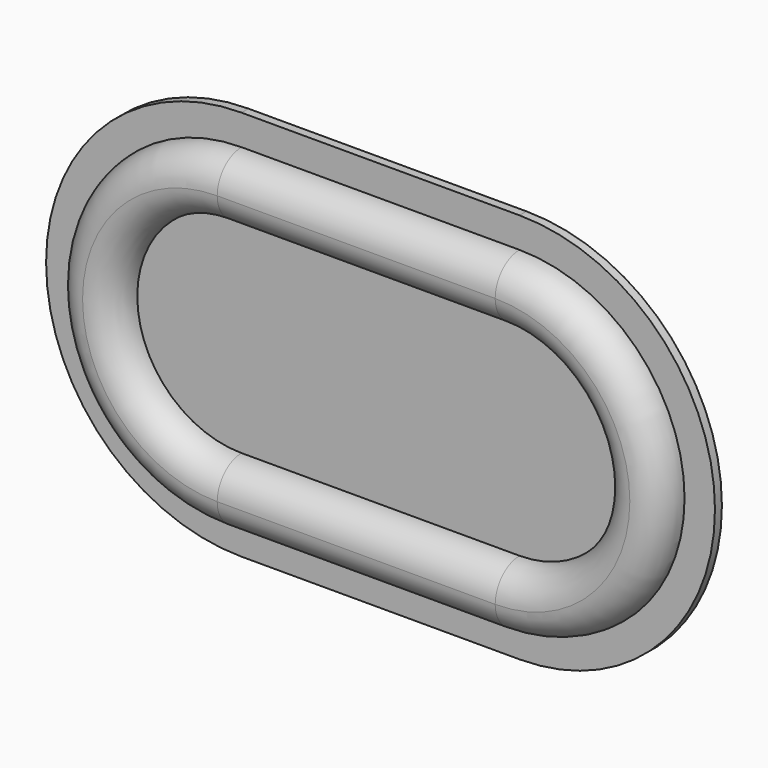
from build123d import *

# Parameters (mm, degrees)
F0_W     = 32
F0_H     = 45
F1_DEPTH = 1
F3_DEPTH = 3.5
F4_R     = 3.49999


# Not quite as in the source:
# - a fillet or chamfer is up to 0.001 mm smaller than in the source, because OpenCascade refuses the exact size


with BuildPart() as f1:
    # F0 (on Front) → F1 (new body)
    with BuildSketch(Plane.XZ):
        with BuildLine():
            Line((16, 22.5), (16, -22.5))
            ThreePointArc((16, -22.5), (38.5, 0), (16, 22.5))
        make_face()
        Rectangle(F0_W, F0_H)
        with BuildLine():
            ThreePointArc((-16, 22.5), (-38.5, 0), (-16, -22.5))
            Line((-16, -22.5), (-16, 22.5))
        make_face()
    extrude(amount=F1_DEPTH)

    # F2 (on face) → F3 (join)
    with BuildSketch(Plane.XZ.offset(1)):
        with BuildLine():
            ThreePointArc((16, -19), (35, 0), (16, 19))
            Line((16, 19), (-16, 19))
            ThreePointArc((-16, 19), (-35, 0), (-16, -19))
            Line((-16, -19), (16, -19))
        make_face()
        with BuildLine():
            ThreePointArc((-16, -12), (-28, 0), (-16, 12))
            Line((-16, 12), (16, 12))
            ThreePointArc((16, 12), (28, 0), (16, -12))
            Line((16, -12), (-16, -12))
        make_face(mode=Mode.SUBTRACT)
    extrude(amount=F3_DEPTH)

    # F4 (radius 3.5 in the source; OpenCascade refuses exactly that, so slightly less here)
    f4_edges = [f1.edges().sort_by_distance(p)[0] for p in [
        (0, -4.5, 19),
        (0, -4.5, 12),
    ]]
    fillet(f4_edges, radius=F4_R)


solid = f1.part
